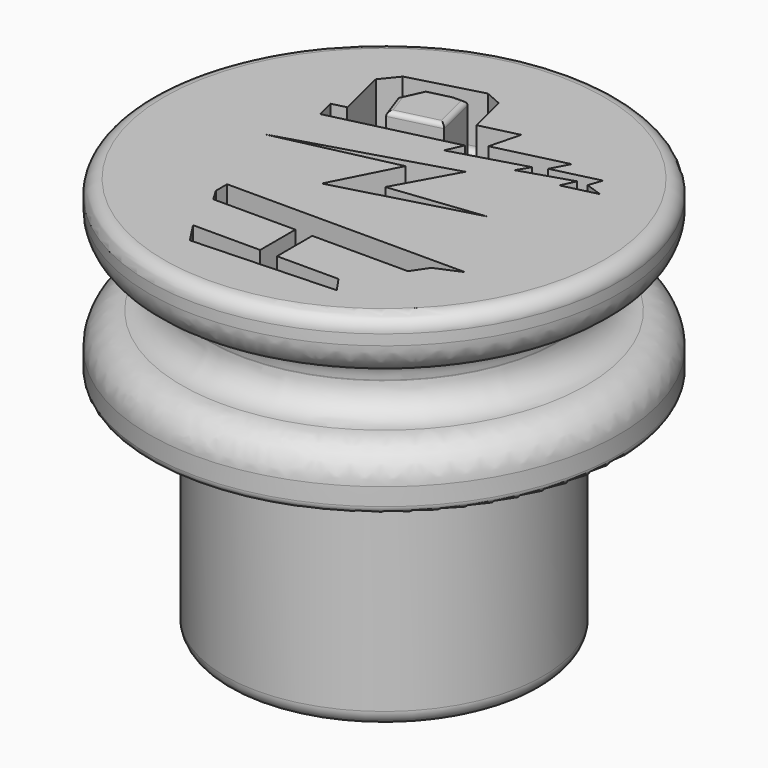
from build123d import *

# Parameters (mm, degrees)
F2_R           = 1.9
F3_R           = 2.1727922061
F4_R           = 0.9656854249
F5_R           = 0.5
F7_DEPTH       = 5.8
F8_R           = 0.1
F9_W           = 1.1126463069
F9_H           = 2.9087299481
F10_DEPTH      = 3.61
F11_R          = 1
F12_R          = 0.2897056275
F13_T1_DEPTH   = 4.4562289253
F13_T3_DEPTH   = 3.2764838258
F13_T5_DEPTH   = 1.9452996333
F13_T7_DEPTH   = 3.4232065966
F13_T9_DEPTH   = 6.77975084
F13_T11_DEPTH  = 3.7270542649
F13_T13_DEPTH  = 3.196072537
F13_T15_DEPTH  = 3.5575258146
F13_T17_DEPTH  = 1.9462715533
F13_T19_DEPTH  = 2.1888564173
F13_T21_DEPTH  = 4.3161100523
F13_T26_DEPTH  = 10.2397508361
F13_T31_DEPTH  = 4.1195166903
F13_T36_DEPTH  = 6.7245550943
F13_T41_DEPTH  = 5.122534233
F13_T46_DEPTH  = 3.3142663971
F13_T51_DEPTH  = 3.0311328749
F13_T56_DEPTH  = 5.4540597414
F13_T61_DEPTH  = 2.9600375429
F13_T66_DEPTH  = 6.9152063996
F13_T71_DEPTH  = 3.2036500019
F13_T77_DEPTH  = 3.2036500019
F13_T81_DEPTH  = 9.2397508361
F13_T88_DEPTH  = 5.4562289253
F13_T92_DEPTH  = 1.9452996333
F13_T99_DEPTH  = 4.5575258146
F13_T103_DEPTH = 4.7270542649
F13_T110_DEPTH = 6.7245550943
F13_T114_DEPTH = 4.1195166903
F13_T121_DEPTH = 5.122534233
F13_T125_DEPTH = 3.3142663971
F13_T132_DEPTH = 3.1888564173
F13_T136_DEPTH = 2.9462715533
F13_T143_DEPTH = 5.4540597414
F13_T147_DEPTH = 3.0311328749
F13_T154_DEPTH = 6.9152063996
F13_T158_DEPTH = 2.9600375429
F14_R          = 0.3


# Not quite as in the source:
# - a fillet or chamfer that OpenCascade refuses, or shapes differently, is made with other operations: its cross-section is extruded or revolved along the edge and cut away or added


with BuildPart() as f1:
    # F0 (on Right) → F1 (revolve)
    with BuildSketch(Plane.YZ):
        Polygon((-15.5, -11.5), (-10.5, -11.5), (-10.5, -26.5), (0, -26.5), (0, 0), (-15.5, 0), (-15.5, -3.83), (-11.5, -3.83), (-11.5, -7.67), (-15.5, -7.67), align=None)
    revolve(axis=Axis((0, 0, -13.25), (0, 0, 1)))

    # F2
    f2_edges = [f1.edges().sort_by_distance(p)[0] for p in [
        (0, 11.5, -3.83),
        (0, 11.5, -7.67),
    ]]
    fillet(f2_edges, radius=F2_R)

    # F3
    f3_edges = [f1.edges().sort_by_distance(p)[0] for p in [
        (0, 15.5, -3.83),
        (0, 15.5, -7.67),
    ]]
    fillet(f3_edges, radius=F3_R)

    # F4
    f4_edges = [f1.edges().sort_by_distance(p)[0] for p in [
        (0, 15.5, 0),
    ]]
    fillet(f4_edges, radius=F4_R)

    # F5
    f5_edges = [f1.edges().sort_by_distance(p)[0] for p in [
        (0, 15.5, -11.5),
    ]]
    fillet(f5_edges, radius=F5_R)

    # F6 (on face) → F7 (cut)
    with BuildSketch(Plane.XY):
        Polygon((2.8064250946, 3.1980199274), (-7.8971497715, 0), (0, 1.7621739535), (-2.1515581063, -2.4433782296), (6.787632592, 0), (0.6449833262, -0.708766599), align=None)
    extrude(amount=-F7_DEPTH, mode=Mode.SUBTRACT)

    # F8
    f8_edges = [f1.edges().sort_by_distance(p)[0] for p in [
        (-1.075779, -0.340602, -5.8),
        (2.318037, -1.221689, -5.8),
        (1.725704, 1.244627, -5.8),
        (3.716308, -0.354383, -5.8),
        (-2.545362, 1.59901, -5.8),
        (-3.948575, 0.881087, -5.8),
    ]]
    fillet(f8_edges, radius=F8_R)

    # F9 (on face) → F10 (cut)
    with BuildSketch(Plane.XY):
        Polygon((7.5338045135, 5.0342432223), (9.7839524969, 5.583059974), (8.6588785052, 5.967231933), (8.9646605922, 6.8627357956), (5.9310551292, 6.1228317944), (6.5459338948, 7.2843912058), (1.955932609, 6.1648783495), (2.4846883025, 8.2173813134), (0, 7.6113595881), (-0.6461925511, 10.2607482252), (-1.7412017332, 10.7419388369), (-6.351263728, 9.4796605408), (-7.2487664848, 8.3751218054), (-6.443046589, 5.0141198962), (-7.3623010542, 4.7937506039), (-7.064725738, 3.5524368286), (0.9480011067, 5.4732966237), (0.4540659138, 4.375662189), (5.1738913171, 5.7477052324), (4.6799560077, 4.924479872), (7.9728569835, 5.967231933), align=None)
        Polygon((-1.3897551676, 6.6941289458), (-4.5950496569, 5.9123495594), (-5.1987483166, 7.6113595881), (-4.5253462032, 9.0950879173), (-2.9485989362, 9.4796605408), (-2.0691533285, 9.4796605408), align=None, mode=Mode.SUBTRACT)
        Polygon((-5.4182750173, -7.3141381145), (0, -7.3141381145), (1.1126463069, -7.3141381145), (7.4240406975, -7.3141381145), (8.1375027075, -6.2713860534), (9.7839524969, -5.5579240434), (-5.9122103266, -5.5579240434), (-5.9122103266, -6.4909127541), align=None)
        with Locations((0.5563231534, -8.7685030885)):
            Rectangle(F9_W, F9_H)
        Polygon((-4.4304043986, -10.2228680626), (-3.4974156879, -11.6497911513), (5.8873533271, -11.2656196579), (5.1738913171, -10.2228680626), (1.1126463069, -10.2228680626), (0, -10.2228680626), align=None)
    extrude(amount=-F10_DEPTH, mode=Mode.SUBTRACT)

    # F11
    f11_edges = [f1.edges().sort_by_distance(p)[0] for p in [
        (0, 10.5, -26.5),
    ]]
    fillet(f11_edges, radius=F11_R)

    # F12
    f12_edges = [f1.edges().sort_by_distance(p)[0] for p in [
        (-2.992402, 6.303239, 0),
        (-1.729454, 8.086895, 0),
        (-2.508876, 9.479661, 0),
        (-3.736973, 9.287374, 0),
        (-4.862047, 8.353224, 0),
        (-4.896899, 6.761855, 0),
        (-4.896899, 6.761855, -3.61),
        (-4.862047, 8.353224, -3.61),
        (-3.736973, 9.287374, -3.61),
        (-2.508876, 9.479661, -3.61),
        (-1.729454, 8.086895, -3.61),
        (-2.992402, 6.303239, -3.61),
    ]]
    fillet(f12_edges, radius=F12_R)

    # F13: fillet of radius 0.4 on 21 edges, made by hand

    # F13_s2 → F13_t1 (join)
    with BuildSketch(Plane(origin=(-2.5256826166, 10.5357012289, 0), x_dir=(0, 0, 1), z_dir=(0.233121102, -0.9724477116, 0))):
        with BuildLine():
            ThreePointArc((-3.61, 4.6966287555), (-3.4928427125, 4.979471468), (-3.21, 5.0966287555))
            Line((-3.21, 5.0966287555), (-3.61, 5.0966287555))
            Line((-3.61, 5.0966287555), (-3.61, 4.6966287555))
        make_face()
    extrude(amount=F13_T1_DEPTH)

    # F13_s4 → F13_t3 (join)
    with BuildSketch(Plane(origin=(-1.7199627208, 7.1746993197, 0), x_dir=(0, 0, 1), z_dir=(0.233121102, -0.9724477116, 0))):
        with BuildLine():
            ThreePointArc((-3.61, 5.6419283888), (-3.4928427125, 5.9247711013), (-3.21, 6.0419283888))
            Line((-3.21, 6.0419283888), (-3.61, 6.0419283888))
            Line((-3.61, 6.0419283888), (-3.61, 5.6419283888))
        make_face()
    extrude(amount=F13_T3_DEPTH)

    # F13_s6 → F13_t5 (join)
    with BuildSketch(Plane(origin=(-4.9562049702, -1.1881317119, 0), x_dir=(0, 0, 1), z_dir=(-0.9724477116, -0.233121102, 0))):
        with BuildLine():
            ThreePointArc((-3.61, 5.9779795397), (-3.4928427125, 6.2608222522), (-3.21, 6.3779795397))
            Line((-3.21, 6.3779795397), (-3.61, 6.3779795397))
            Line((-3.61, 6.3779795397), (-3.61, 5.9779795397))
        make_face()
    extrude(amount=F13_T5_DEPTH)

    # F13_s8 → F13_t7 (join)
    with BuildSketch(Plane(origin=(2.7443645329, 3.3774346739, 0), x_dir=(0, 0, 1), z_dir=(-0.6306201496, -0.7760916357, 0))):
        with BuildLine():
            ThreePointArc((-3.61, 10.5072276034), (-3.4928427125, 10.7900703158), (-3.21, 10.9072276034))
            Line((-3.21, 10.9072276034), (-3.61, 10.9072276034))
            Line((-3.61, 10.9072276034), (-3.61, 10.5072276034))
        make_face()
    extrude(amount=F13_T7_DEPTH)

    # F13_s10 → F13_t9 (join)
    with BuildSketch(Plane(origin=(2.0808460979, 0.5697552158, 0), x_dir=(0, 0, 1), z_dir=(-0.964498391, -0.2640887231, 0))):
        with BuildLine():
            ThreePointArc((-3.61, 10.4204144673), (-3.4928427125, 10.7032571798), (-3.21, 10.8204144673))
            Line((-3.21, 10.8204144673), (-3.61, 10.8204144673))
            Line((-3.61, 10.8204144673), (-3.61, 10.4204144673))
        make_face()
    extrude(amount=F13_T9_DEPTH)

    # F13_s12 → F13_t11 (join)
    with BuildSketch(Plane(origin=(-1.7521944363, 7.1839949588, 0), x_dir=(0, 0, 1), z_dir=(-0.2369562496, 0.9715203218, 0))):
        with BuildLine():
            ThreePointArc((-3.61, 1.4035592225), (-3.4928427125, 1.686401935), (-3.21, 1.8035592225))
            Line((-3.21, 1.8035592225), (-3.61, 1.8035592225))
            Line((-3.61, 1.8035592225), (-3.61, 1.4035592225))
        make_face()
    extrude(amount=F13_T11_DEPTH)

    # F13_s14 → F13_t13 (join)
    with BuildSketch(Plane(origin=(-3.4052922264, 1.4964209213, 0), x_dir=(0, 0, 1), z_dir=(-0.9155039919, 0.4023088874, 0))):
        with BuildLine():
            ThreePointArc((-3.61, 8.7337869533), (-3.4928427125, 9.0166296658), (-3.21, 9.1337869533))
            Line((-3.21, 9.1337869533), (-3.61, 9.1337869533))
            Line((-3.61, 9.1337869533), (-3.61, 8.7337869533))
        make_face()
    extrude(amount=F13_T13_DEPTH)

    # F13_s16 → F13_t15 (join)
    with BuildSketch(Plane(origin=(5.2084030607, 1.2703426043, 0), x_dir=(0, 0, 1), z_dir=(-0.9715203218, -0.2369562496, 0))):
        with BuildLine():
            ThreePointArc((-3.61, 6.9945905168), (-3.4928427125, 7.2774332292), (-3.21, 7.3945905168))
            Line((-3.21, 7.3945905168), (-3.61, 7.3945905168))
            Line((-3.61, 7.3945905168), (-3.61, 6.9945905168))
        make_face()
    extrude(amount=F13_T15_DEPTH)

    # F13_s18 → F13_t17 (join)
    with BuildSketch(Plane(origin=(2.7290019105, 7.9920696991, 0), x_dir=(0, 0, 1), z_dir=(0.3231441185, 0.9463497655, 0))):
        with BuildLine():
            ThreePointArc((-3.61, 5.8660517399), (-3.4928427125, 6.1488944524), (-3.21, 6.2660517399))
            Line((-3.21, 6.2660517399), (-3.61, 6.2660517399))
            Line((-3.61, 6.2660517399), (-3.61, 5.8660517399))
        make_face()
    extrude(amount=F13_T17_DEPTH)

    # F13_s20 → F13_t19 (join)
    with BuildSketch(Plane(origin=(8.0013003519, -2.7321538436, 0), x_dir=(0, 0, 1), z_dir=(-0.9463497655, 0.3231441185, 0))):
        with BuildLine():
            ThreePointArc((-3.61, 8.0451542025), (-3.4928427125, 8.3279969149), (-3.21, 8.4451542025))
            Line((-3.21, 8.4451542025), (-3.61, 8.4451542025))
            Line((-3.61, 8.4451542025), (-3.61, 8.0451542025))
        make_face()
    extrude(amount=F13_T19_DEPTH)

    # F13_s22 → F13_t21 (join)
    with BuildSketch(Plane(origin=(7.2981962619, 1.7800484213, 0), x_dir=(0, 0, 1), z_dir=(0.9715203218, 0.2369562496, 0))):
        with BuildLine():
            ThreePointArc((-3.61, -3.5056875328), (-3.4928427125, -3.2228448203), (-3.21, -3.1056875328))
            Line((-3.21, -3.1056875328), (-3.61, -3.1056875328))
            Line((-3.61, -3.1056875328), (-3.61, -3.5056875328))
        make_face()
    extrude(amount=F13_T21_DEPTH)


with BuildPart() as f13_tool24:
    # F13_s25 → F13_t26 (new body)
    with BuildSketch(Plane(origin=(-6.847907147, -1.6416221062, 0), x_dir=(0, 0, 1), z_dir=(0.9724477116, 0.233121102, 0))):
        with BuildLine():
            ThreePointArc((-3.61, -5.5014957139), (-3.4928427125, -5.2186530015), (-3.21, -5.1014957139))
            Line((-3.21, -5.1014957139), (-3.61, -5.1014957139))
            Line((-3.61, -5.1014957139), (-3.61, -5.5014957139))
        make_face()
    extrude(amount=F13_T26_DEPTH)

    split(bisect_by=Plane(origin=(-1.2598596069, 0.5669364757, 0), x_dir=(0, 0, 1), z_dir=(-0.9119215993, 0.4103644682, 0)), keep=Keep.TOP)


with BuildPart() as f1_1:
    add(f1.part)

    # F13_t23: union F13_tool24
    add(f13_tool24.part)


with BuildPart() as f13_tool29:
    # F13_s30 → F13_t31 (new body)
    with BuildSketch(Plane(origin=(1.3615837013, 5.285341826, 0), x_dir=(0, 0, 1), z_dir=(0.2494699362, 0.9683825437, 0))):
        with BuildLine():
            ThreePointArc((-3.61, -0.0438608132), (-3.4928427125, 0.2389818992), (-3.21, 0.3561391868))
            Line((-3.21, 0.3561391868), (-3.61, 0.3561391868))
            Line((-3.61, 0.3561391868), (-3.61, -0.0438608132))
        make_face()
    extrude(amount=F13_T31_DEPTH)

    split(bisect_by=Plane(origin=(-1.3093809345, 5.3684601648, 0), x_dir=(0, 0, 1), z_dir=(-0.2369562496, 0.9715203218, 0)), keep=Keep.TOP)


with BuildPart() as f1_2:
    add(f1_1.part)

    # F13_t28: union F13_tool29
    add(f13_tool29.part)


with BuildPart() as f13_tool34:
    # F13_s35 → F13_t36 (new body)
    with BuildSketch(Plane(origin=(8.8268351511, 2.1528872905, 0), x_dir=(0, 0, 1), z_dir=(-0.9715203218, -0.2369562496, 0))):
        with BuildLine():
            ThreePointArc((-3.61, 5.1258341427), (-3.4928427125, 5.4086768552), (-3.21, 5.5258341427))
            Line((-3.21, 5.5258341427), (-3.61, 5.5258341427))
            Line((-3.61, 5.5258341427), (-3.61, 5.1258341427))
        make_face()
    extrude(amount=F13_T36_DEPTH)

    split(bisect_by=Plane(origin=(0.3448789716, -0.0888460202, 0), x_dir=(0, 0, 1), z_dir=(0.9683825437, -0.2494699362, 0)), keep=Keep.TOP)


with BuildPart() as f1_3:
    add(f1_2.part)

    # F13_t33: union F13_tool34
    add(f13_tool34.part)


with BuildPart() as f13_tool39:
    # F13_s40 → F13_t41 (new body)
    with BuildSketch(Plane(origin=(11.0126861734, 2.6860218517, 0), x_dir=(0, 0, 1), z_dir=(-0.9715203218, -0.2369562496, 0))):
        with BuildLine():
            ThreePointArc((-3.61, 4.1430549359), (-3.4928427125, 4.4258976483), (-3.21, 4.5430549359))
            Line((-3.21, 4.5430549359), (-3.61, 4.5430549359))
            Line((-3.61, 4.5430549359), (-3.61, 4.1430549359))
        make_face()
    extrude(amount=F13_T41_DEPTH)

    split(bisect_by=Plane(origin=(2.1011230445, -1.1122426726, 0), x_dir=(0, 0, 1), z_dir=(0.8838081944, -0.4678494155, 0)), keep=Keep.TOP)


with BuildPart() as f1_4:
    add(f1_3.part)

    # F13_t38: union F13_tool39
    add(f13_tool39.part)


with BuildPart() as f13_tool44:
    # F13_s45 → F13_t46 (new body)
    with BuildSketch(Plane(origin=(3.3620826692, 6.3512662727, 0), x_dir=(0, 0, 1), z_dir=(0.4678494155, 0.8838081944, 0))):
        with BuildLine():
            ThreePointArc((-3.61, 1.9773518484), (-3.4928427125, 2.2601945609), (-3.21, 2.3773518484))
            Line((-3.21, 2.3773518484), (-3.61, 2.3773518484))
            Line((-3.61, 2.3773518484), (-3.61, 1.9773518484))
        make_face()
    extrude(amount=F13_T46_DEPTH)

    split(bisect_by=Plane(origin=(-1.0765052594, 4.4136701935, 0), x_dir=(0, 0, 1), z_dir=(-0.2369562496, 0.9715203218, 0)), keep=Keep.TOP)


with BuildPart() as f1_5:
    add(f1_4.part)

    # F13_t43: union F13_tool44
    add(f13_tool44.part)


with BuildPart() as f13_tool49:
    # F13_s50 → F13_t51 (new body)
    with BuildSketch(Plane(origin=(4.1702811468, 8.8618684463, 0), x_dir=(0, 0, 1), z_dir=(-0.4257962099, -0.9048190911, 0))):
        with BuildLine():
            ThreePointArc((-3.61, -5.0731684688), (-3.4928427125, -4.7903257564), (-3.21, -4.6731684688))
            Line((-3.21, -4.6731684688), (-3.61, -4.6731684688))
            Line((-3.61, -4.6731684688), (-3.61, -5.0731684688))
        make_face()
    extrude(amount=F13_T51_DEPTH)

    split(bisect_by=Plane(origin=(-0.99077078, 3.1287495755, 0), x_dir=(0, 0, 1), z_dir=(0.3018917272, -0.9533422182, 0)), keep=Keep.TOP)


with BuildPart() as f1_6:
    add(f1_5.part)

    # F13_t48: union F13_tool49
    add(f13_tool49.part)


with BuildPart() as f13_tool54:
    # F13_s55 → F13_t56 (new body)
    with BuildSketch(Plane(origin=(4.7173845695, 1.4938385693, 0), x_dir=(0, 0, 1), z_dir=(0.9533422182, 0.3018917272, 0))):
        with BuildLine():
            ThreePointArc((-3.61, -3.6818745626), (-3.4928427125, -3.3990318501), (-3.21, -3.2818745626))
            Line((-3.21, -3.2818745626), (-3.61, -3.2818745626))
            Line((-3.61, -3.2818745626), (-3.61, -3.6818745626))
        make_face()
    extrude(amount=F13_T56_DEPTH)

    split(bisect_by=Plane(origin=(4.2283720466, -1.9898174222, 0), x_dir=(0, 0, 1), z_dir=(-0.9048190911, 0.4257962099, 0)), keep=Keep.TOP)


with BuildPart() as f1_7:
    add(f1_6.part)

    # F13_t53: union F13_tool54
    add(f13_tool54.part)


with BuildPart() as f13_tool59:
    # F13_s60 → F13_t61 (new body)
    with BuildSketch(Plane(origin=(4.4198082062, 7.3663456214, 0), x_dir=(0, 0, 1), z_dir=(-0.5144958268, -0.8574928829, 0))):
        with BuildLine():
            ThreePointArc((-3.61, -1.8794046259), (-3.4928427125, -1.5965619134), (-3.21, -1.4794046259))
            Line((-3.21, -1.4794046259), (-3.61, -1.4794046259))
            Line((-3.61, -1.4794046259), (-3.61, -1.8794046259))
        make_face()
    extrude(amount=F13_T61_DEPTH)

    split(bisect_by=Plane(origin=(-1.1374999003, 3.9129974468, 0), x_dir=(0, 0, 1), z_dir=(0.2791425083, -0.9602496863, 0)), keep=Keep.TOP)


with BuildPart() as f1_8:
    add(f1_7.part)

    # F13_t58: union F13_tool59
    add(f13_tool59.part)


with BuildPart() as f13_tool64:
    # F13_s65 → F13_t66 (new body)
    with BuildSketch(Plane(origin=(0.6313161278, 0.1835222338, 0), x_dir=(0, 0, 1), z_dir=(0.9602496863, 0.2791425083, 0))):
        with BuildLine():
            ThreePointArc((-3.61, -4.4749791462), (-3.4928427125, -4.1921364337), (-3.21, -4.0749791462))
            Line((-3.21, -4.0749791462), (-3.61, -4.0749791462))
            Line((-3.61, -4.0749791462), (-3.61, -4.4749791462))
        make_face()
    extrude(amount=F13_T66_DEPTH)

    split(bisect_by=Plane(origin=(1.2685789377, -0.7611475061, 0), x_dir=(0, 0, 1), z_dir=(-0.8574928829, 0.5144958268, 0)), keep=Keep.TOP)


with BuildPart() as f1_9:
    add(f1_8.part)

    # F13_t63: union F13_tool64
    add(f13_tool64.part)


with BuildPart() as f13_tool69:
    # F13_s70 → F13_t71 (new body)
    with BuildSketch(Plane(origin=(2.6182251818, 5.8182817473, 0), x_dir=(0, 0, 1), z_dir=(-0.4103644682, -0.9119215993, 0))):
        with BuildLine():
            ThreePointArc((-3.61, 0.9815437729), (-3.4928427125, 1.2643864854), (-3.21, 1.3815437729))
            Line((-3.21, 1.3815437729), (-3.61, 1.3815437729))
            Line((-3.61, 1.3815437729), (-3.61, 0.9815437729))
        make_face()
    extrude(amount=F13_T71_DEPTH)

    split(bisect_by=Plane(origin=(-1.1892663026, 4.9609378328, 0), x_dir=(0, 0, 1), z_dir=(0.233121102, -0.9724477116, 0)), keep=Keep.TOP)


with BuildPart() as f1_10:
    add(f1_9.part)

    # F13_t68: union F13_tool69
    add(f13_tool69.part)


with BuildPart() as f13_tool75:
    # F13_s76 → F13_t77 (new body)
    with BuildSketch(Plane(origin=(2.6182251818, 5.8182817473, 0), x_dir=(0, 0, 1), z_dir=(-0.4103644682, -0.9119215993, 0))):
        with BuildLine():
            ThreePointArc((-3.61, 0.9815437729), (-3.4928427125, 1.2643864854), (-3.21, 1.3815437729))
            Line((-3.21, 1.3815437729), (-3.61, 1.3815437729))
            Line((-3.61, 1.3815437729), (-3.61, 0.9815437729))
        make_face()
    extrude(amount=F13_T77_DEPTH)

    split(bisect_by=Plane(origin=(-1.1892663026, 4.9609378328, 0), x_dir=(0, 0, 1), z_dir=(-0.233121102, 0.9724477116, 0)), keep=Keep.TOP)


with BuildPart() as f13_tool79:
    # F13_s80 → F13_t81 (new body)
    with BuildSketch(Plane(origin=(-5.8754594354, -1.4085010042, 0), x_dir=(0, 0, 1), z_dir=(0.9724477116, 0.233121102, 0))):
        with BuildLine():
            ThreePointArc((-3.61, -5.5014957139), (-3.4928427125, -5.2186530015), (-3.21, -5.1014957139))
            Line((-3.21, -5.1014957139), (-3.61, -5.1014957139))
            Line((-3.61, -5.1014957139), (-3.61, -5.5014957139))
        make_face()
    extrude(amount=F13_T81_DEPTH)

    split(bisect_by=Plane(origin=(-1.2598596069, 0.5669364757, 0), x_dir=(0, 0, 1), z_dir=(0.9119215993, -0.4103644682, 0)), keep=Keep.TOP)


with BuildPart() as f13_tool75_1:
    add(f13_tool75.part)

    # F13_t83: intersect F13_tool79
    add(f13_tool79.part, mode=Mode.INTERSECT)


with BuildPart() as f1_11:
    add(f1_10.part)

    # F13_t73: union F13_tool75
    add(f13_tool75_1.part)


with BuildPart() as f13_tool86:
    # F13_s87 → F13_t88 (new body)
    with BuildSketch(Plane(origin=(-2.5256826166, 10.5357012289, 0), x_dir=(0, 0, 1), z_dir=(0.233121102, -0.9724477116, 0))):
        with BuildLine():
            ThreePointArc((-3.61, 4.6966287555), (-3.4928427125, 4.979471468), (-3.21, 5.0966287555))
            Line((-3.21, 5.0966287555), (-3.61, 5.0966287555))
            Line((-3.61, 5.0966287555), (-3.61, 4.6966287555))
        make_face()
    extrude(amount=F13_T88_DEPTH)

    split(bisect_by=Plane(origin=(-1.4868416188, 6.2022516081, 0), x_dir=(0, 0, 1), z_dir=(0.233121102, -0.9724477116, 0)), keep=Keep.TOP)


with BuildPart() as f13_tool90:
    # F13_s91 → F13_t92 (new body)
    with BuildSketch(Plane(origin=(-3.9837572586, -0.9550106099, 0), x_dir=(0, 0, 1), z_dir=(-0.9724477116, -0.233121102, 0))):
        with BuildLine():
            ThreePointArc((-3.61, 5.9779795397), (-3.4928427125, 6.2608222522), (-3.21, 6.3779795397))
            Line((-3.21, 6.3779795397), (-3.61, 6.3779795397))
            Line((-3.61, 6.3779795397), (-3.61, 5.9779795397))
        make_face()
    extrude(amount=F13_T92_DEPTH)

    split(bisect_by=Plane(origin=(-4.9562049702, -1.1881317119, 0), x_dir=(0, 0, 1), z_dir=(0.9724477116, 0.233121102, 0)), keep=Keep.TOP)


with BuildPart() as f13_tool86_1:
    add(f13_tool86.part)

    # F13_t94: intersect F13_tool90
    add(f13_tool90.part, mode=Mode.INTERSECT)


with BuildPart() as f1_12:
    add(f1_11.part)

    # F13_t84: union F13_tool86
    add(f13_tool86_1.part)


with BuildPart() as f13_tool97:
    # F13_s98 → F13_t99 (new body)
    with BuildSketch(Plane(origin=(5.2084030607, 1.2703426043, 0), x_dir=(0, 0, 1), z_dir=(-0.9715203218, -0.2369562496, 0))):
        with BuildLine():
            ThreePointArc((-3.61, 6.9945905168), (-3.4928427125, 7.2774332292), (-3.21, 7.3945905168))
            Line((-3.21, 7.3945905168), (-3.61, 7.3945905168))
            Line((-3.61, 7.3945905168), (-3.61, 6.9945905168))
        make_face()
    extrude(amount=F13_T99_DEPTH)

    split(bisect_by=Plane(origin=(1.7521944363, 0.4273646293, 0), x_dir=(0, 0, 1), z_dir=(-0.9715203218, -0.2369562496, 0)), keep=Keep.TOP)


with BuildPart() as f13_tool101:
    # F13_s102 → F13_t103 (new body)
    with BuildSketch(Plane(origin=(-1.5152381867, 6.212474637, 0), x_dir=(0, 0, 1), z_dir=(-0.2369562496, 0.9715203218, 0))):
        with BuildLine():
            ThreePointArc((-3.61, 1.4035592225), (-3.4928427125, 1.686401935), (-3.21, 1.8035592225))
            Line((-3.21, 1.8035592225), (-3.61, 1.8035592225))
            Line((-3.61, 1.8035592225), (-3.61, 1.4035592225))
        make_face()
    extrude(amount=F13_T103_DEPTH)

    split(bisect_by=Plane(origin=(-1.7521944363, 7.1839949588, 0), x_dir=(0, 0, 1), z_dir=(0.2369562496, -0.9715203218, 0)), keep=Keep.TOP)


with BuildPart() as f13_tool97_1:
    add(f13_tool97.part)

    # F13_t105: intersect F13_tool101
    add(f13_tool101.part, mode=Mode.INTERSECT)


with BuildPart() as f1_13:
    add(f1_12.part)

    # F13_t95: union F13_tool97
    add(f13_tool97_1.part)


with BuildPart() as f13_tool108:
    # F13_s109 → F13_t110 (new body)
    with BuildSketch(Plane(origin=(8.8268351511, 2.1528872905, 0), x_dir=(0, 0, 1), z_dir=(-0.9715203218, -0.2369562496, 0))):
        with BuildLine():
            ThreePointArc((-3.61, 5.1258341427), (-3.4928427125, 5.4086768552), (-3.21, 5.5258341427))
            Line((-3.21, 5.5258341427), (-3.61, 5.5258341427))
            Line((-3.61, 5.5258341427), (-3.61, 5.1258341427))
        make_face()
    extrude(amount=F13_T110_DEPTH)

    split(bisect_by=Plane(origin=(0.3448789716, -0.0888460202, 0), x_dir=(0, 0, 1), z_dir=(-0.9683825437, 0.2494699362, 0)), keep=Keep.TOP)


with BuildPart() as f13_tool112:
    # F13_s113 → F13_t114 (new body)
    with BuildSketch(Plane(origin=(1.3615837013, 5.285341826, 0), x_dir=(0, 0, 1), z_dir=(0.2494699362, 0.9683825437, 0))):
        with BuildLine():
            ThreePointArc((-3.61, -0.0438608132), (-3.4928427125, 0.2389818992), (-3.21, 0.3561391868))
            Line((-3.21, 0.3561391868), (-3.61, 0.3561391868))
            Line((-3.61, 0.3561391868), (-3.61, -0.0438608132))
        make_face()
    extrude(amount=F13_T114_DEPTH)

    split(bisect_by=Plane(origin=(-1.3093809345, 5.3684601648, 0), x_dir=(0, 0, 1), z_dir=(0.2369562496, -0.9715203218, 0)), keep=Keep.TOP)


with BuildPart() as f13_tool108_1:
    add(f13_tool108.part)

    # F13_t116: intersect F13_tool112
    add(f13_tool112.part, mode=Mode.INTERSECT)


with BuildPart() as f1_14:
    add(f1_13.part)

    # F13_t106: union F13_tool108
    add(f13_tool108_1.part)


with BuildPart() as f13_tool119:
    # F13_s120 → F13_t121 (new body)
    with BuildSketch(Plane(origin=(11.0126861734, 2.6860218517, 0), x_dir=(0, 0, 1), z_dir=(-0.9715203218, -0.2369562496, 0))):
        with BuildLine():
            ThreePointArc((-3.61, 4.1430549359), (-3.4928427125, 4.4258976483), (-3.21, 4.5430549359))
            Line((-3.21, 4.5430549359), (-3.61, 4.5430549359))
            Line((-3.61, 4.5430549359), (-3.61, 4.1430549359))
        make_face()
    extrude(amount=F13_T121_DEPTH)

    split(bisect_by=Plane(origin=(2.1011230445, -1.1122426726, 0), x_dir=(0, 0, 1), z_dir=(-0.8838081944, 0.4678494155, 0)), keep=Keep.TOP)


with BuildPart() as f13_tool123:
    # F13_s124 → F13_t125 (new body)
    with BuildSketch(Plane(origin=(3.3620826692, 6.3512662727, 0), x_dir=(0, 0, 1), z_dir=(0.4678494155, 0.8838081944, 0))):
        with BuildLine():
            ThreePointArc((-3.61, 1.9773518484), (-3.4928427125, 2.2601945609), (-3.21, 2.3773518484))
            Line((-3.21, 2.3773518484), (-3.61, 2.3773518484))
            Line((-3.61, 2.3773518484), (-3.61, 1.9773518484))
        make_face()
    extrude(amount=F13_T125_DEPTH)

    split(bisect_by=Plane(origin=(-1.0765052594, 4.4136701935, 0), x_dir=(0, 0, 1), z_dir=(0.2369562496, -0.9715203218, 0)), keep=Keep.TOP)


with BuildPart() as f13_tool119_1:
    add(f13_tool119.part)

    # F13_t127: intersect F13_tool123
    add(f13_tool123.part, mode=Mode.INTERSECT)


with BuildPart() as f1_15:
    add(f1_14.part)

    # F13_t117: union F13_tool119
    add(f13_tool119_1.part)


with BuildPart() as f13_tool130:
    # F13_s131 → F13_t132 (new body)
    with BuildSketch(Plane(origin=(8.0013003519, -2.7321538436, 0), x_dir=(0, 0, 1), z_dir=(-0.9463497655, 0.3231441185, 0))):
        with BuildLine():
            ThreePointArc((-3.61, 8.0451542025), (-3.4928427125, 8.3279969149), (-3.21, 8.4451542025))
            Line((-3.21, 8.4451542025), (-3.61, 8.4451542025))
            Line((-3.61, 8.4451542025), (-3.61, 8.0451542025))
        make_face()
    extrude(amount=F13_T132_DEPTH)

    split(bisect_by=Plane(origin=(5.9298765947, -2.0248377661, 0), x_dir=(0, 0, 1), z_dir=(-0.9463497655, 0.3231441185, 0)), keep=Keep.TOP)


with BuildPart() as f13_tool134:
    # F13_s135 → F13_t136 (new body)
    with BuildSketch(Plane(origin=(2.405857792, 7.0457199336, 0), x_dir=(0, 0, 1), z_dir=(0.3231441185, 0.9463497655, 0))):
        with BuildLine():
            ThreePointArc((-3.61, 5.8660517399), (-3.4928427125, 6.1488944524), (-3.21, 6.2660517399))
            Line((-3.21, 6.2660517399), (-3.61, 6.2660517399))
            Line((-3.61, 6.2660517399), (-3.61, 5.8660517399))
        make_face()
    extrude(amount=F13_T136_DEPTH)

    split(bisect_by=Plane(origin=(2.7290019105, 7.9920696991, 0), x_dir=(0, 0, 1), z_dir=(-0.3231441185, -0.9463497655, 0)), keep=Keep.TOP)


with BuildPart() as f13_tool130_1:
    add(f13_tool130.part)

    # F13_t138: intersect F13_tool134
    add(f13_tool134.part, mode=Mode.INTERSECT)


with BuildPart() as f1_16:
    add(f1_15.part)

    # F13_t128: union F13_tool130
    add(f13_tool130_1.part)


with BuildPart() as f13_tool141:
    # F13_s142 → F13_t143 (new body)
    with BuildSketch(Plane(origin=(4.7173845695, 1.4938385693, 0), x_dir=(0, 0, 1), z_dir=(0.9533422182, 0.3018917272, 0))):
        with BuildLine():
            ThreePointArc((-3.61, -3.6818745626), (-3.4928427125, -3.3990318501), (-3.21, -3.2818745626))
            Line((-3.21, -3.2818745626), (-3.61, -3.2818745626))
            Line((-3.61, -3.2818745626), (-3.61, -3.6818745626))
        make_face()
    extrude(amount=F13_T143_DEPTH)

    split(bisect_by=Plane(origin=(4.2283720466, -1.9898174222, 0), x_dir=(0, 0, 1), z_dir=(0.9048190911, -0.4257962099, 0)), keep=Keep.TOP)


with BuildPart() as f13_tool145:
    # F13_s146 → F13_t147 (new body)
    with BuildSketch(Plane(origin=(4.1702811468, 8.8618684463, 0), x_dir=(0, 0, 1), z_dir=(-0.4257962099, -0.9048190911, 0))):
        with BuildLine():
            ThreePointArc((-3.61, -5.0731684688), (-3.4928427125, -4.7903257564), (-3.21, -4.6731684688))
            Line((-3.21, -4.6731684688), (-3.61, -4.6731684688))
            Line((-3.61, -4.6731684688), (-3.61, -5.0731684688))
        make_face()
    extrude(amount=F13_T147_DEPTH)

    split(bisect_by=Plane(origin=(-0.99077078, 3.1287495755, 0), x_dir=(0, 0, 1), z_dir=(-0.3018917272, 0.9533422182, 0)), keep=Keep.TOP)


with BuildPart() as f13_tool141_1:
    add(f13_tool141.part)

    # F13_t149: intersect F13_tool145
    add(f13_tool145.part, mode=Mode.INTERSECT)


with BuildPart() as f1_17:
    add(f1_16.part)

    # F13_t139: union F13_tool141
    add(f13_tool141_1.part)


with BuildPart() as f13_tool152:
    # F13_s153 → F13_t154 (new body)
    with BuildSketch(Plane(origin=(0.6313161278, 0.1835222338, 0), x_dir=(0, 0, 1), z_dir=(0.9602496863, 0.2791425083, 0))):
        with BuildLine():
            ThreePointArc((-3.61, -4.4749791462), (-3.4928427125, -4.1921364337), (-3.21, -4.0749791462))
            Line((-3.21, -4.0749791462), (-3.61, -4.0749791462))
            Line((-3.61, -4.0749791462), (-3.61, -4.4749791462))
        make_face()
    extrude(amount=F13_T154_DEPTH)

    split(bisect_by=Plane(origin=(1.2685789377, -0.7611475061, 0), x_dir=(0, 0, 1), z_dir=(0.8574928829, -0.5144958268, 0)), keep=Keep.TOP)


with BuildPart() as f13_tool156:
    # F13_s157 → F13_t158 (new body)
    with BuildSketch(Plane(origin=(4.4198082062, 7.3663456214, 0), x_dir=(0, 0, 1), z_dir=(-0.5144958268, -0.8574928829, 0))):
        with BuildLine():
            ThreePointArc((-3.61, -1.8794046259), (-3.4928427125, -1.5965619134), (-3.21, -1.4794046259))
            Line((-3.21, -1.4794046259), (-3.61, -1.4794046259))
            Line((-3.61, -1.4794046259), (-3.61, -1.8794046259))
        make_face()
    extrude(amount=F13_T158_DEPTH)

    split(bisect_by=Plane(origin=(-1.1374999003, 3.9129974468, 0), x_dir=(0, 0, 1), z_dir=(-0.2791425083, 0.9602496863, 0)), keep=Keep.TOP)


with BuildPart() as f13_tool152_1:
    add(f13_tool152.part)

    # F13_t160: intersect F13_tool156
    add(f13_tool156.part, mode=Mode.INTERSECT)


with BuildPart() as f1_18:
    add(f1_17.part)

    # F13_t150: union F13_tool152
    add(f13_tool152_1.part)

    # F14
    f14_edges = [f1_18.edges().sort_by_distance(p)[0] for p in [
        (-2.709138, -7.314138, -3.61),
        (0, -8.768503, -3.61),
        (-3.96391, -10.93633, -3.61),
        (-2.215202, -10.222868, -3.61),
        (1.194969, -11.457705, -3.61),
        (5.530622, -10.744244, -3.61),
        (3.143269, -10.222868, -3.61),
        (1.112646, -8.768503, -3.61),
        (4.268344, -7.314138, -3.61),
        (7.780772, -6.792762, -3.61),
        (8.960728, -5.914655, -3.61),
        (1.935871, -5.557924, -3.61),
        (-5.665243, -6.902525, -3.61),
        (-5.91221, -6.024418, -3.61),
    ]]
    fillet(f14_edges, radius=F14_R)


solid = f1_18.part
